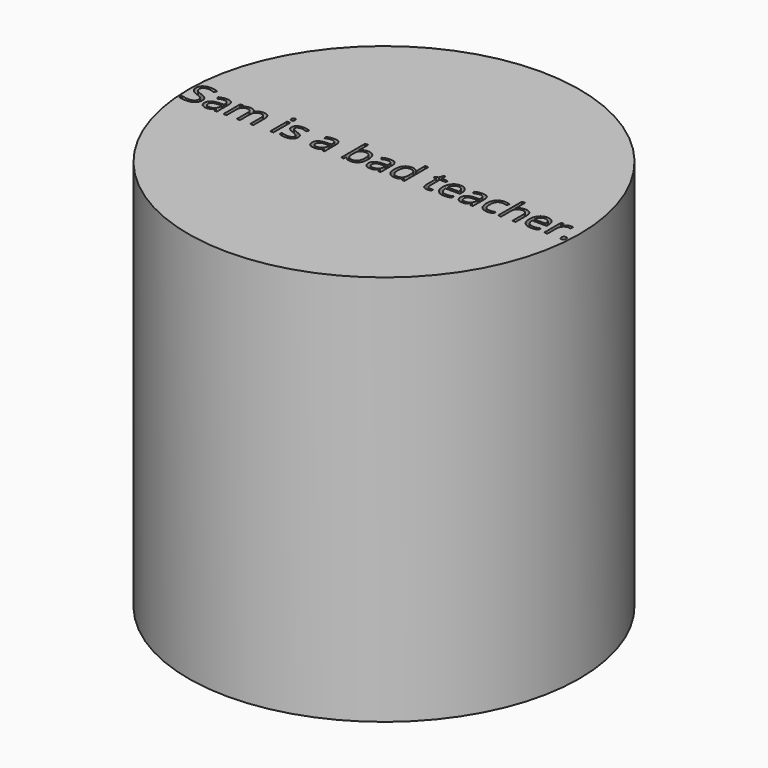
from build123d import *

# Parameters (mm, degrees)
F0_R         = 38.1
F1_DEPTH     = 76.2
F2_TEXT_SIZE = 7.6578492939
F3_DEPTH     = 5.08


# Not quite as in the source:
# - Text() gives the source's letters only with a copy of the font that has no kerning and outlines rounded to 1/6400 em; it was checked with that copy


with BuildPart() as f1:
    # F0 (on Top) → F1 (new body)
    with BuildSketch(Plane.XY):
        Circle(F0_R)
    extrude(amount=F1_DEPTH)

    # F2 (on face) → F3 (cut)
    with BuildSketch(Plane.XY.offset(76.2)):
        with Locations((-38.0152390496, -2.9736514916)):
            Text('Sam is a bad teacher.', F2_TEXT_SIZE, font='Open Sans', text_align=(TextAlign.LEFT, TextAlign.BOTTOM))
    extrude(amount=-F3_DEPTH, mode=Mode.SUBTRACT)


solid = f1.part
